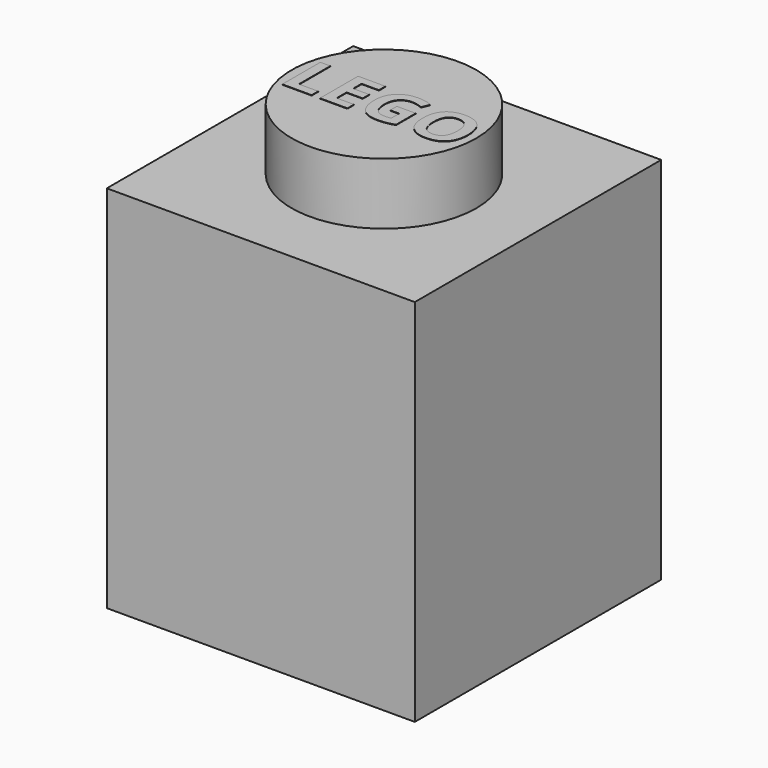
from build123d import *

# Parameters (mm, degrees)
F0_W         = 8
F0_H         = 8
F1_DEPTH     = 9.6
F2_W         = 4.8
F2_H         = 4.8
F3_DEPTH     = 8
F4_R         = 1.6
F5_DEPTH     = 1.6
F6_R         = 2.4
F6_R_2       = 1.6
F7_DEPTH     = 1.6
F8_TEXT_SIZE = 1.7347239408
F9_DEPTH     = 0.01


# Not quite as in the source:
# - Text() gives the source's letters only with a copy of the font that has no kerning and outlines rounded to 1/6400 em; it was checked with that copy


with BuildPart() as f1:
    # F0 (on Top) → F1 (new body)
    with BuildSketch(Plane.XY):
        Rectangle(F0_W, F0_H)
    extrude(amount=F1_DEPTH)

    # F2 (on face) → F3 (cut)
    with BuildSketch(Plane(origin=(0, 0, 0), x_dir=(1, 0, 0), z_dir=(0, 0, -1))):
        Rectangle(F2_W, F2_H)
    extrude(amount=-F3_DEPTH, mode=Mode.SUBTRACT)

    # F4 (on face) → F5 (cut)
    with BuildSketch(Plane.XY.offset(9.6)):
        Circle(F4_R)
    extrude(amount=-F5_DEPTH, mode=Mode.SUBTRACT)

    # F6 (on face) → F7 (join)
    with BuildSketch(Plane.XY.offset(9.6)):
        Circle(F6_R)
        Circle(F6_R_2, mode=Mode.SUBTRACT)
        Circle(F6_R_2)
    extrude(amount=F7_DEPTH)

    # F8 (on face) → F9 (join)
    with BuildSketch(Plane.XY.offset(11.2)):
        with Locations((-2.3, -0.6245012374)):
            Text('LEGO', F8_TEXT_SIZE, font='Open Sans', font_style=FontStyle.BOLD, text_align=(TextAlign.LEFT, TextAlign.BOTTOM))
    extrude(amount=F9_DEPTH)


solid = f1.part
